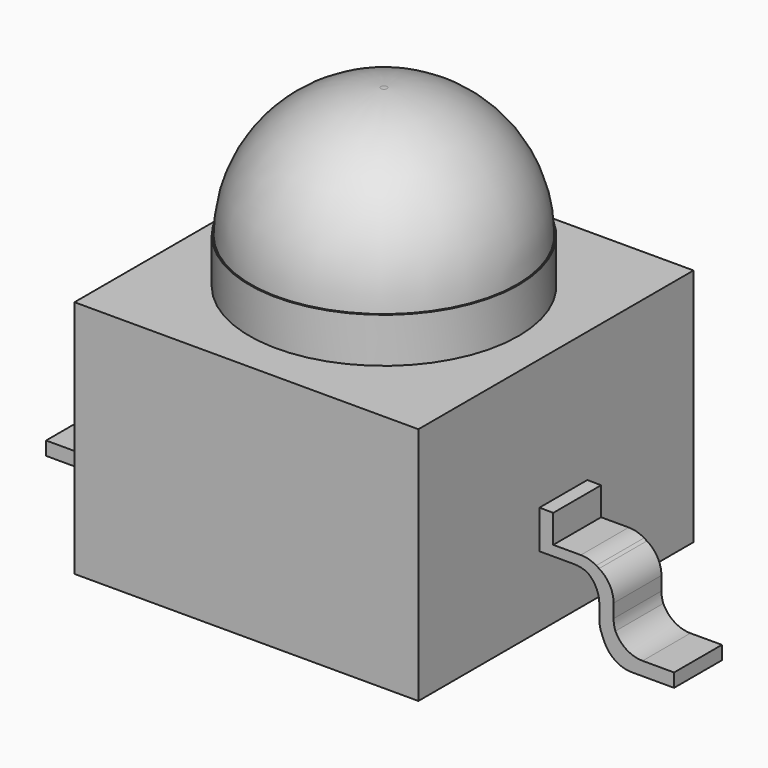
from build123d import *

# Parameters (mm, degrees)
F0_W         = 2.3
F0_H         = 2.3
F1_DEPTH     = 1.6
F2_R         = 0.9
F3_DEPTH     = 0.3
F4_R         = 0.89
F5_DEPTH     = 0.87
F6_R         = 0.86999
F8_DEPTH     = 0.2
F9_R         = 0.2
F10_T1_DEPTH = 0.4


# Not quite as in the source:
# - a fillet or chamfer that OpenCascade refuses, or shapes differently, is made with other operations: its cross-section is extruded or revolved along the edge and cut away or added
# - a fillet or chamfer is up to 0.001 mm smaller than in the source, because OpenCascade refuses the exact size


with BuildPart() as f1:
    # F0 (on Top) → F1 (new body)
    with BuildSketch(Plane.XY):
        Rectangle(F0_W, F0_H)
    extrude(amount=F1_DEPTH)

    # F2 (on face) → F3 (join)
    with BuildSketch(Plane.XY.offset(1.6)):
        Circle(F2_R)
    extrude(amount=F3_DEPTH)


with BuildPart() as f5:
    # F4 (on face) → F5 (new body)
    with BuildSketch(Plane.XY.offset(1.9)):
        Circle(F4_R)
    extrude(amount=F5_DEPTH)

    # F6 (radius 0.87 in the source; OpenCascade refuses exactly that, so slightly less here)
    f6_edges = [f5.edges().sort_by_distance(p)[0] for p in [
        (-0.89, 0, 2.77),
    ]]
    fillet(f6_edges, radius=F6_R)


with BuildPart() as f8:
    # F7 (on Front) → F8 (new body, symmetric)
    with BuildSketch(Plane.XZ):
        Polygon((-1.2000221869, 0.5113023705), (-1.2000221869, 0.7686837657), (-1.2919139418, 0.7676174894), (-1.2919139418, 0.5792069319), (-1.5315959482, 0.5792069319), (-1.6954116582, 0.4809875769), (-1.6954116582, 0.2360437474), (-1.756004122, 0.0907330487), (-2.1, 0.0907330487), (-2.1, 0), (-1.683620195, 0), (-1.6002507828, 0.199933569), (-1.6002507828, 0.4406041371), (-1.4906145475, 0.5113023705), align=None)
    extrude(amount=F8_DEPTH, both=True)

    # F9
    f9_edges = [f8.edges().sort_by_distance(p)[0] for p in [
        (-1.695412, 0, 0.480988),
        (-1.531596, 0, 0.579207),
        (-1.600251, 0, 0.199934),
        (-1.68362, 0, 0),
    ]]
    fillet(f9_edges, radius=F9_R)

    # F10: fillet of radius 0.2 on 4 edges, made by hand

    # F10_s2 → F10_t1 (join)
    with BuildSketch(Plane.XZ.offset(-0.2)):
        with BuildLine():
            ThreePointArc((-1.8892982143, 0.0907330487), (-1.7783807823, 0.1243079205), (-1.7047037359, 0.2137598158))
            Line((-1.7047037359, 0.2137598158), (-1.756004122, 0.0907330487))
            Line((-1.756004122, 0.0907330487), (-1.8892982143, 0.0907330487))
        make_face()
        with BuildLine():
            ThreePointArc((-1.7108171798, 0.1990987714), (-1.6993008532, 0.2368221359), (-1.6954116582, 0.2760720043))
            Line((-1.6954116582, 0.2760720043), (-1.6954116582, 0.2360437474))
            Line((-1.6954116582, 0.2360437474), (-1.7108171798, 0.1990987714))
        make_face()
        with BuildLine():
            ThreePointArc((-1.6002507828, 0.3315961203), (-1.5758604852, 0.4273104473), (-1.5086384588, 0.4996797652))
            Line((-1.5086384588, 0.4996797652), (-1.6002507828, 0.4406041371))
            Line((-1.6002507828, 0.4406041371), (-1.6002507828, 0.3315961203))
        make_face()
        with BuildLine():
            ThreePointArc((-1.540109264, 0.4793860154), (-1.4882161497, 0.5031574316), (-1.4317215879, 0.5113023705))
            Line((-1.4317215879, 0.5113023705), (-1.4906145475, 0.5113023705))
            Line((-1.4906145475, 0.5113023705), (-1.540109264, 0.4793860154))
        make_face()
    extrude(amount=F10_T1_DEPTH)


with BuildPart() as f11_1:
    # F11: instance of F8
    add(f8.part.mirror(Plane.YZ))


solid = Compound([f1.part, f5.part, f8.part, f11_1.part])
